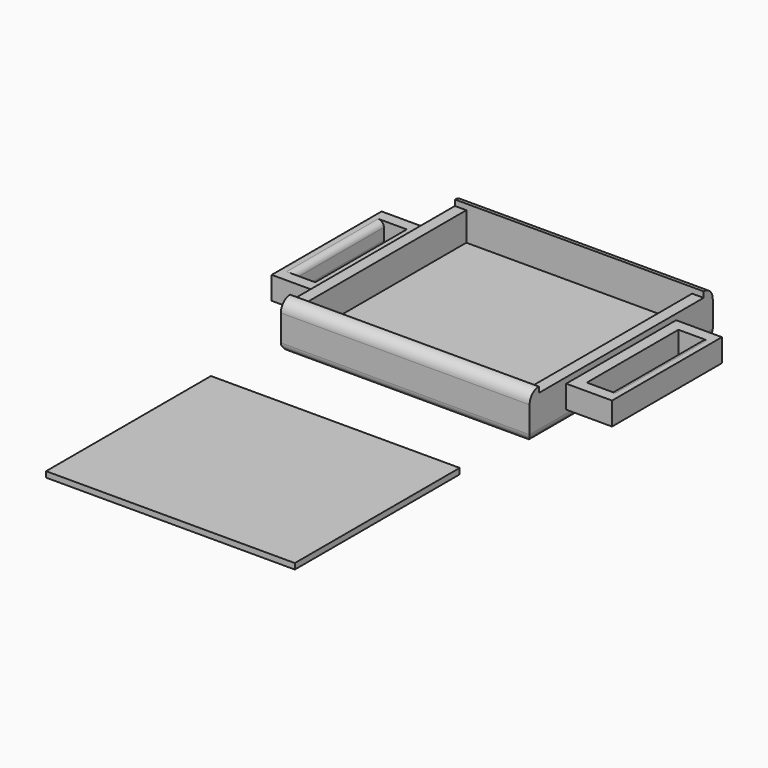
from build123d import *

# Parameters (mm, degrees)
F0_W      = 55.1858954132
F0_H      = 50.8
F1_DEPTH  = 10.16
F2_W      = 30.48
F2_H      = 5.08
F3_DEPTH  = 10.16
F4_W      = 30.48
F4_H      = 5.08
F5_DEPTH  = 10.16
F6_W      = 50.1058954132
F6_H      = 45.72
F7_DEPTH  = 7.62
F8_R      = 2.53999
F9_W      = 2.54
F9_H      = 45.72
F10_DEPTH = 1.27
F11_W     = 55.1942
F11_H     = 45.72
F12_DEPTH = 1.27
F13_W     = 5.08
F13_H     = 25.4
F14_DEPTH = 25.4
F15_R     = 1.27
F16_R     = 1.778


# Not quite as in the source:
# - a fillet or chamfer is up to 0.001 mm smaller than in the source, because OpenCascade refuses the exact size


with BuildPart() as f1:
    # F0 (on Top) → F1 (new body)
    with BuildSketch(Plane.XY):
        with Locations((1.2412052602, 12.0331741214)):
            Rectangle(F0_W, F0_H)
    extrude(amount=F1_DEPTH)

    # F2 (on face) → F3 (join)
    with BuildSketch(Plane.YZ.offset(28.8341529667)):
        with Locations((12.0331741214, 5.08)):
            Rectangle(F2_W, F2_H)
    extrude(amount=F3_DEPTH)

    # F4 (on face) → F5 (join)
    with BuildSketch(Plane(origin=(-26.3517424464, 0, 0), x_dir=(0, -1, 0), z_dir=(-1, 0, 0))):
        with Locations((-12.0331741214, 5.08)):
            Rectangle(F4_W, F4_H)
    extrude(amount=F5_DEPTH)

    # F6 (on face) → F7 (cut)
    with BuildSketch(Plane.XY.offset(10.16)):
        with Locations((1.2412052602, 12.0331741214)):
            Rectangle(F6_W, F6_H)
    extrude(amount=-F7_DEPTH, mode=Mode.SUBTRACT)

    # F8 (radius 2.54 in the source; OpenCascade refuses exactly that, so slightly less here)
    f8_edges = [f1.edges().sort_by_distance(p)[0] for p in [
        (1.241205, -13.366826, 10.16),
        (1.241205, 37.433174, 10.16),
    ]]
    fillet(f8_edges, radius=F8_R)

    # F9 (on face) → F10 (cut)
    with BuildSketch(Plane.XY.offset(10.16)):
        with Locations((27.5641529667, 12.0331741214)):
            Rectangle(F9_W, F9_H)
        with Locations((-25.0817424464, 12.0331741214)):
            Rectangle(F9_W, F9_H)
    extrude(amount=-F10_DEPTH, mode=Mode.SUBTRACT)

    # F13 (on face) → F14 (cut)
    with BuildSketch(Plane.XY.offset(7.62)):
        with Locations((-31.4317424464, 12.0331741214)):
            Rectangle(F13_W, F13_H)
        with Locations((33.9141529667, 12.0331741214)):
            Rectangle(F13_W, F13_H)
    extrude(amount=-F14_DEPTH, mode=Mode.SUBTRACT)

    # F15
    f15_edges = [f1.edges().sort_by_distance(p)[0] for p in [
        (-33.971742, 12.033174, 7.62),
        (-33.971742, 12.033174, 2.54),
        (36.454153, 12.033174, 2.54),
        (36.454153, 12.033174, 7.62),
    ]]
    fillet(f15_edges, radius=F15_R)

    # F16
    f16_edges = [f1.edges().sort_by_distance(p)[0] for p in [
        (28.834153, 12.033174, 0),
        (1.241205, 37.433174, 0),
        (-26.351742, 12.033174, 0),
        (1.241205, -13.366826, 0),
    ]]
    fillet(f16_edges, radius=F16_R)


with BuildPart() as f12:
    # F11 (on Top) → F12 (new body)
    with BuildSketch(Plane.XY):
        with Locations((-1.0460983113, -52.7580435419)):
            Rectangle(F11_W, F11_H)
    extrude(amount=F12_DEPTH)


solid = Compound([f1.part, f12.part])
